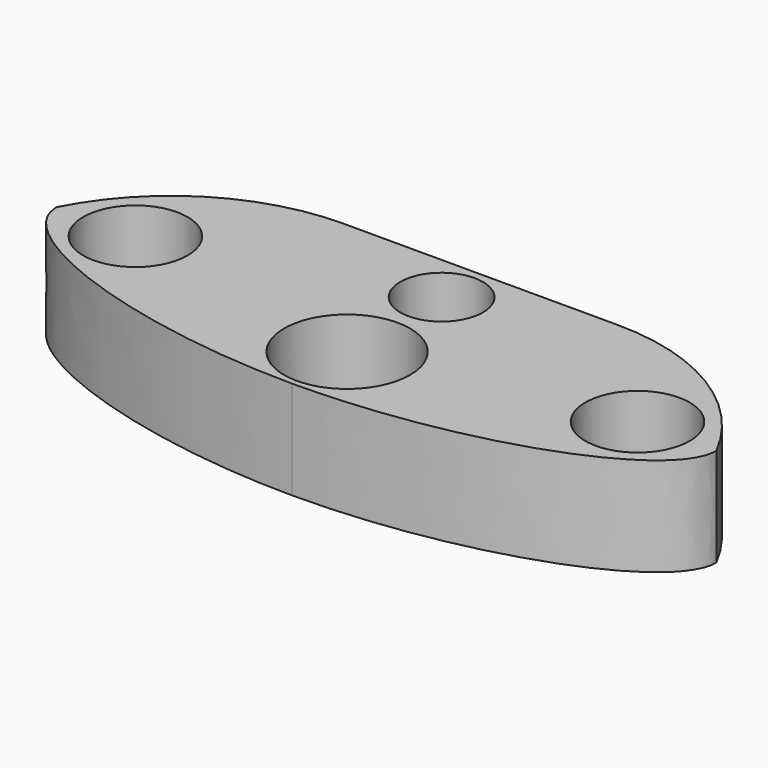
from build123d import *

# Parameters (mm, degrees)
F0_W        = 335
F0_H        = 120
F0_R        = 26.5
F0_R_2      = 32
F0_R_3      = 21
F1_DEPTH    = 50
F3_DEPTH    = 60
F4_T1_DEPTH = 539.8979480904
F4_T3_DEPTH = 539.8979491671


# Not quite as in the source:
# - a fillet or chamfer that OpenCascade refuses, or shapes differently, is made with other operations: its cross-section is extruded or revolved along the edge and cut away or added


with BuildPart() as f1:
    # F0 (on Top) → F1 (new body)
    with BuildSketch(Plane.XY):
        with Locations((1.7180761695, 76.1685734987)):
            Rectangle(F0_W, F0_H)
        with Locations((-125.7819238305, 76.1685734987)):
            Circle(F0_R, mode=Mode.SUBTRACT)
        with Locations((1.7180761695, 51.1685734987)):
            Circle(F0_R_2, mode=Mode.SUBTRACT)
        with Locations((129.2180761695, 76.1685734987)):
            Circle(F0_R, mode=Mode.SUBTRACT)
        with Locations((1.7180761695, 111.1685734987)):
            Circle(F0_R_3, mode=Mode.SUBTRACT)
    extrude(amount=F1_DEPTH)

    # F2 (on face) → F3 (cut)
    with BuildSketch(Plane.XY.offset(50)):
        with BuildLine():
            Line((-165.7819238305, 16.1685734987), (1.7180761695, 16.1685734987))
            add(Edge.make_bspline(
                [(1.7180761695, 16.1685734987), (-82.0319238305, 16.1685734987), (-165.7819235634, 46.168573403), (-165.7819238305, 76.1685733073)],
                knots=[0, 0, 0, 0, 0.25, 0.25, 0.25, 0.25], degree=3))
            Line((-165.7819238305, 76.1685732116), (-165.7819238305, 16.1685734987))
        make_face()
        with BuildLine():
            add(Edge.make_bspline(
                [(169.2180761695, 76.1685736449), (169.2180763735, 46.1685735718), (85.4680761695, 16.1685734987), (1.7180761695, 16.1685734987)],
                knots=[0.75, 0.75, 0.75, 0.75, 1, 1, 1, 1], degree=3))
            Line((1.7180761695, 16.1685734987), (169.2180761695, 16.1685734987))
            Line((169.2180761695, 16.1685734987), (169.2180761695, 76.168573718))
        make_face()
    extrude(amount=-F3_DEPTH, mode=Mode.SUBTRACT)

    # F4: fillet of radius 110 on 2 edges, made by hand

    # F4_s2 → F4_t1 (cut)
    with BuildSketch(Plane.XY.offset(-244.9489740452)):
        with BuildLine():
            ThreePointArc((71.2384865514, 136.1685734987), (128.6841129293, 119.9768887488), (169.2180761695, 76.1685736814))
            Line((169.2180761695, 76.1685736814), (169.2180761695, 136.1685734987))
            Line((169.2180761695, 136.1685734987), (71.2384865514, 136.1685734987))
        make_face()
    extrude(amount=F4_T1_DEPTH, mode=Mode.SUBTRACT)

    # F4_s4 → F4_t3 (cut)
    with BuildSketch(Plane.XY.offset(-244.9489745835)):
        with BuildLine():
            ThreePointArc((-67.8023339971, 136.1685734987), (-125.247960577, 119.9768886251), (-165.7819238305, 76.1685732595))
            Line((-165.7819238305, 76.1685732595), (-165.7819238305, 136.1685734987))
            Line((-165.7819238305, 136.1685734987), (-67.8023339971, 136.1685734987))
        make_face()
    extrude(amount=F4_T3_DEPTH, mode=Mode.SUBTRACT)


solid = f1.part
